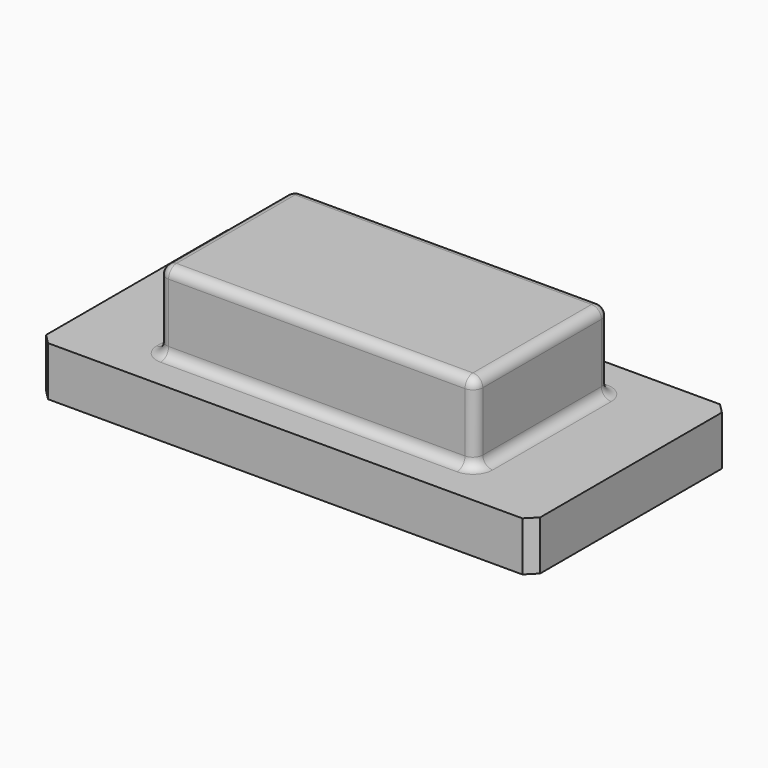
from build123d import *

# Parameters (mm, degrees)
F0_W     = 500
F0_H     = 250
F1_DEPTH = 25
F2_W     = 320
F2_H     = 170
F3_DEPTH = 80
F4_R     = 10
F5_SIZE  = 10


with BuildPart() as f1:
    # F0 (on Top) → F1 (new body, symmetric)
    with BuildSketch(Plane.XY):
        Rectangle(F0_W, F0_H)
    extrude(amount=F1_DEPTH, both=True)

    # F2 (on face) → F3 (join)
    with BuildSketch(Plane.XY.offset(25)):
        Rectangle(F2_W, F2_H)
    extrude(amount=F3_DEPTH)

    # F4
    f4_edges = [f1.edges().sort_by_distance(p)[0] for p in [
        (0, -85, 105),
        (160, 0, 105),
        (0, 85, 105),
        (-160, 0, 105),
        (-160, -85, 65),
        (160, -85, 65),
        (160, 85, 65),
        (-160, 85, 65),
        (-160, 0, 25),
        (0, -85, 25),
        (160, 0, 25),
        (0, 85, 25),
    ]]
    fillet(f4_edges, radius=F4_R)

    # F5
    f5_edges = [f1.edges().sort_by_distance(p)[0] for p in [
        (-250, -125, 0),
        (-250, 125, 0),
        (250, 125, 0),
        (250, -125, 0),
    ]]
    chamfer(f5_edges, length=F5_SIZE)


solid = f1.part
